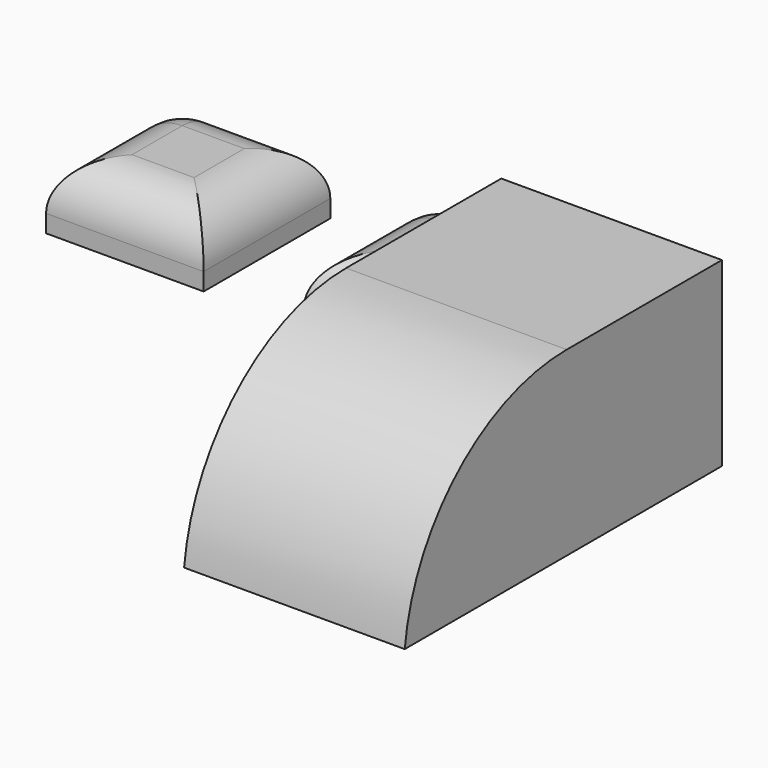
from build123d import *

# Parameters (mm, degrees)
F0_W        = 107.1967259049
F0_H        = 107.7348701656
F1_DEPTH    = 44.45
F2_R        = 32.5001429767
F4_W        = 269.7381898761
F4_H        = 123.4003640711
F5_DEPTH    = 150.114
F6_T1_DEPTH = 838.8693310434


# Not quite as in the source:
# - a fillet or chamfer that OpenCascade refuses, or shapes differently, is made with other operations: its cross-section is extruded or revolved along the edge and cut away or added


with BuildPart() as f1:
    # F0 (on Top) → F1 (new body)
    with BuildSketch(Plane.XY):
        with Locations((-4.3046809733, 13.598324731)):
            Rectangle(F0_W, F0_H)
    extrude(amount=F1_DEPTH)

    # F2
    f2_edges = [f1.edges().sort_by_distance(p)[0] for p in [
        (-57.903044, 67.46576, 22.225),
        (-4.304681, 67.46576, 44.45),
        (-57.903044, 13.598325, 44.45),
        (-4.304681, -40.26911, 44.45),
        (49.293682, 13.598325, 44.45),
    ]]
    fillet(f2_edges, radius=F2_R)


with BuildPart() as f3_1:
    # F3: copy of F1
    add(f1.part.moved(Location((-175.26, 0, 0))))


with BuildPart() as f1_1:
    add(f1.part)

    # F4 (on Right) → F5 (join)
    with BuildSketch(Plane.YZ):
        with Locations((-79.4771648943, 8.0686341971)):
            Rectangle(F4_W, F4_H)
    extrude(amount=F5_DEPTH)

    # F6: fillet of radius 138.5855153345 on 1 edges, made by hand

    # F6_s2 → F6_t1 (cut)
    with BuildSketch(Plane.YZ.offset(-344.3776655217)):
        with BuildLine():
            ThreePointArc((-76.5951936237, 69.7688162327), (-169.0654673533, 34.4072978025), (-214.3462598324, -53.6315478384))
            Line((-214.3462598324, -53.6315478384), (-214.3462598324, 69.7688162327))
            Line((-214.3462598324, 69.7688162327), (-76.5951936237, 69.7688162327))
        make_face()
    extrude(amount=F6_T1_DEPTH, mode=Mode.SUBTRACT)


solid = Compound([f3_1.part, f1_1.part])
